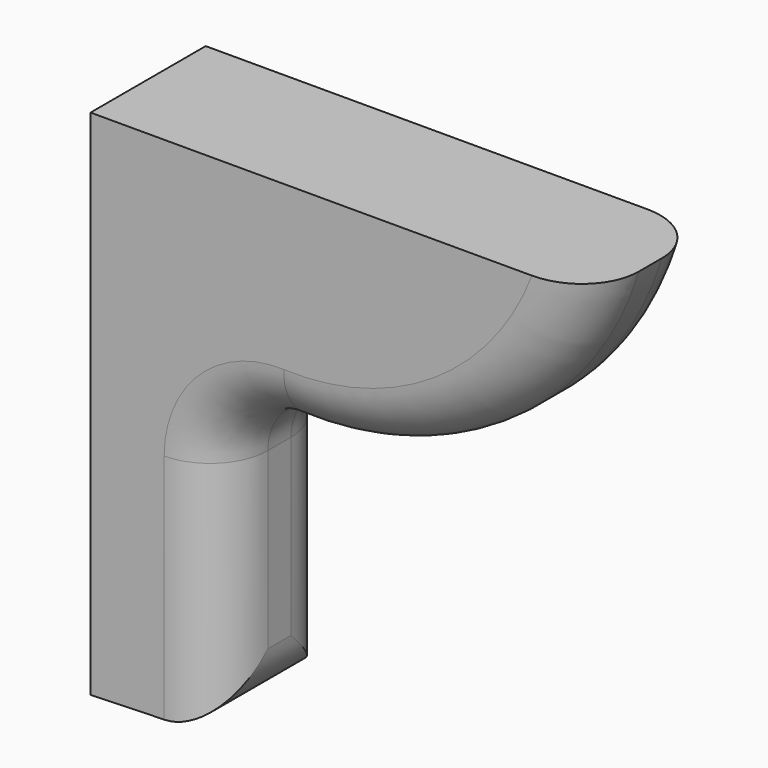
from build123d import *

# Parameters (mm, degrees)
F1_DEPTH = 3.175
F2_F1_R  = 2.54
F2_F2_R  = 2.54


with BuildPart() as f1:
    # F0 (on Front) → F1 (new body, symmetric)
    with BuildSketch(Plane.XZ):
        with BuildLine():
            Line((13.3350007236, 17.7493449301), (-3.0348624568, 17.7493449301))
            Line((-3.0348624568, 17.7493449301), (-3.0348624568, 8.3688618615))
            ThreePointArc((-3.0348624568, 8.3688618615), (7.007326367, 9.8180073261), (13.3350007236, 17.7493449301))
        make_face()
        Polygon((-3.0348624568, 8.3688618615), (-3.0348624568, 17.7493449301), (-8.8243288919, 17.7493449301), (-8.8243288919, -4.8698359169), (-3.0348624568, -4.6902415343), align=None)
    extrude(amount=F1_DEPTH, both=True)

    # F2: fillet of radius 2.54 on 4 edges, made by hand

    # F2_f1
    f2_f1_edges = [f1.edges().sort_by_distance(p)[0] for p in [
        (-3.0348624568, 0, 8.3688618615),
    ]]
    fillet(f2_f1_edges, radius=F2_F1_R)

    # F2_f2
    f2_f2_edges = [f1.edges().sort_by_distance(p)[0] for p in [
        (-3.0348624568, 3.175, 0.3884883664),
        (-3.0348624568, -3.175, 0.3884883664),
        (-3.0348624568, 0, -4.6902415343),
        (-2.2547093843, -3.175, 7.2987582727),
        (-2.2547093843, 3.175, 7.2987582727),
    ]]
    fillet(f2_f2_edges, radius=F2_F2_R)


solid = f1.part
